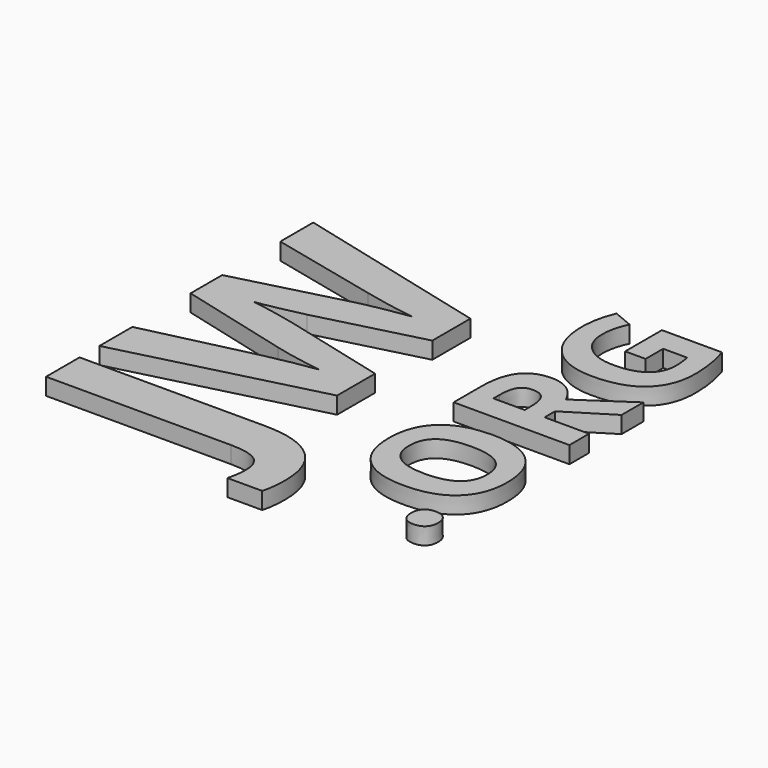
from build123d import *

# Parameters (mm, degrees)
F0_TEXT_SIZE   = 65.4372816655
F0_TEXT_SIZE_2 = 38.3793558751
F1_DEPTH       = 4


# Not quite as in the source:
# - Text() gives the source's letters only with a copy of the font that has no kerning and outlines rounded to 1/6400 em; it was checked with that copy


with BuildPart() as f1:
    # F0 (on Top) → F1 (new body)
    with BuildSketch(Plane.XY):
        with Locations(Location((0, -47.0177093342), (0, 0, 90))):
            Text('JW', F0_TEXT_SIZE, font='Open Sans', font_style=FontStyle.BOLD, text_align=(TextAlign.LEFT, TextAlign.BOTTOM))
        with Locations(Location((45.9161045765, -47.0177093342), (0, 0, 90))):
            Text('.ORG', F0_TEXT_SIZE_2, font='Open Sans', font_style=FontStyle.BOLD, text_align=(TextAlign.LEFT, TextAlign.BOTTOM))
    extrude(amount=-F1_DEPTH)


solid = f1.part
